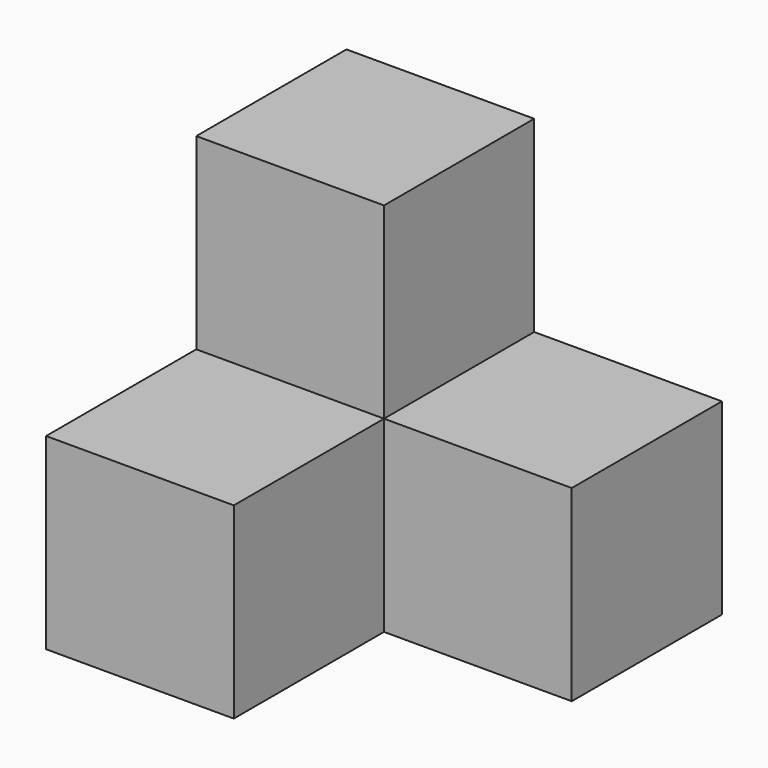
from build123d import *

# Parameters (mm, degrees)
F1_W     = 50.8
F1_H     = 50.8
F2_DEPTH = 25.4
F3_W     = 25.4
F3_H     = 25.4
F4_DEPTH = 25.4
F5_W     = 25.4
F5_H     = 25.4
F6_DEPTH = 25.4


# Not quite as in the source:
# - a variable given as a bare number and used for a length is read in inches; the dataset says mm whatever the document's units were


with BuildPart() as f2:
    # F1 (on Top) → F2 (new body)
    with BuildSketch(Plane.XY):
        Rectangle(F1_W, F1_H)
    extrude(amount=F2_DEPTH)

    # F3 (on face) → F4 (cut)
    with BuildSketch(Plane.XY.offset(25.4)):
        with Locations((12.7, -12.7)):
            Rectangle(F3_W, F3_H)
    extrude(amount=-F4_DEPTH, mode=Mode.SUBTRACT)

    # F5 (on face) → F6 (join)
    with BuildSketch(Plane.XY.offset(25.4)):
        with Locations((-12.7, 12.7)):
            Rectangle(F5_W, F5_H)
    extrude(amount=F6_DEPTH)


solid = f2.part
